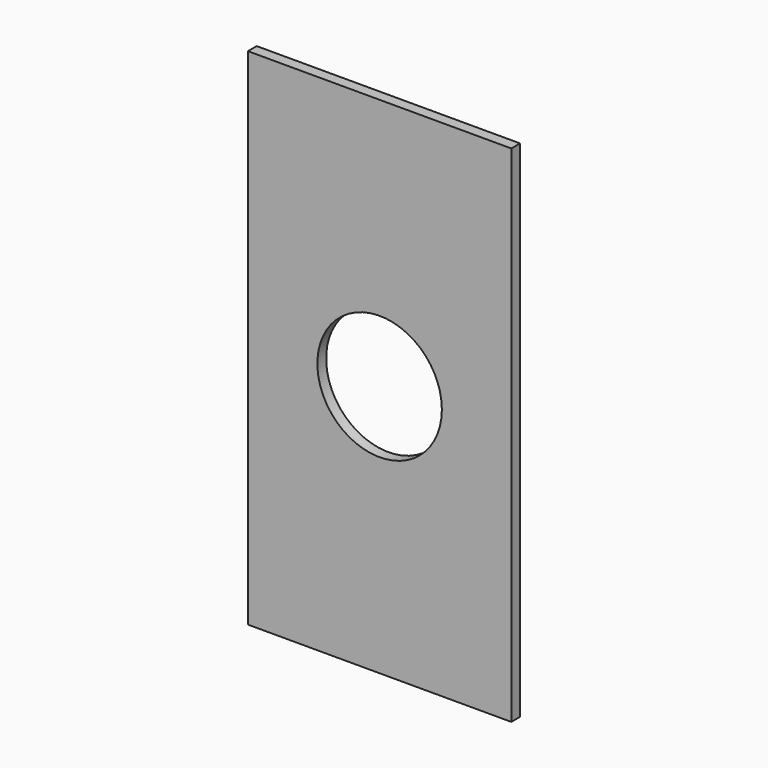
from build123d import *

# Parameters (mm, degrees)
F0_W     = 38.1
F0_H     = 73.025
F1_DEPTH = 1.5875
F2_R     = 9.0043
F3_DEPTH = 25.4


# Not quite as in the source:
# - a length typed as a fraction of an inch, garbled in the dataset ("3 / 203.2 mm" for 3/8 in), is restored


with BuildPart() as f1:
    # F0 (on Front) → F1 (new body)
    with BuildSketch(Plane.XZ):
        Rectangle(F0_W, F0_H)
    extrude(amount=F1_DEPTH)

    # F2 (on face) → F3 (cut)
    with BuildSketch(Plane.XZ.offset(1.5875)):
        Circle(F2_R)
    extrude(amount=-F3_DEPTH, mode=Mode.SUBTRACT)


solid = f1.part
